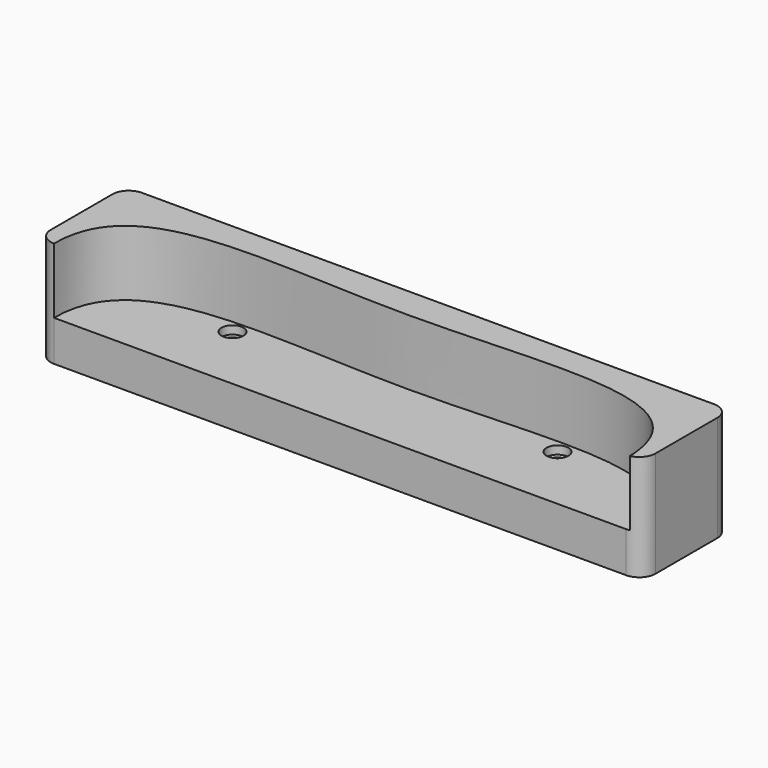
from build123d import *

# Parameters (mm, degrees)
F1_DEPTH = 32.4
F3_DEPTH = 20
F4_R     = 3.35
F5_DEPTH = 2.5
F6_R     = 1.93
F7_DEPTH = 25
F8_R     = 1.93
F9_DEPTH = 25


# Not quite as in the source:
# - a feature names something its author has since deleted; it is built from what else it names


with BuildPart() as f1:
    # F0 (on Top) → F1 (new body)
    with BuildSketch(Plane.XY):
        with BuildLine():
            Line((85.6374964118, -7.5007802074), (-89.3625035882, -7.5007802074))
            ThreePointArc((-89.3625035882, -7.5007802074), (-92.8980374941, -8.9652463014), (-94.3625035882, -12.5007802074))
            Line((-94.3625035882, -12.5007802074), (-94.3625035882, -36.1007802074))
            ThreePointArc((-94.3625035882, -36.1007802074), (-92.8980374941, -39.6363141133), (-89.3625035882, -41.1007802074))
            add(Edge.make_bspline(
                [(-89.3625035882, -41.1007802074), (-59.4269413323, -34.6411043009), (-0.064704069, -1.5309018726), (57.2335608059, -34.7243234216), (85.6374964118, -41.1007802074)],
                knots=[0, 0, 0, 0, 0.5049781057, 1, 1, 1, 1], degree=3))
            ThreePointArc((85.6374964118, -41.1007802074), (89.1730303177, -39.6363141133), (90.6374964118, -36.1007802074))
            Line((90.6374964118, -36.1007802074), (90.6374964118, -12.5007802074))
            ThreePointArc((90.6374964118, -12.5007802074), (89.1730303177, -8.9652463014), (85.6374964118, -7.5007802074))
        make_face()
        with BuildLine():
            add(Edge.make_bspline(
                [(-89.3625035882, -41.1007802074), (-59.4269413323, -34.6411043009), (-0.064704069, -1.5309018726), (57.2335608059, -34.7243234216), (85.6374964118, -41.1007802074)],
                knots=[0, 0, 0, 0, 0.5049781057, 1, 1, 1, 1], degree=3))
            Line((-89.3625035882, -41.1007802074), (85.6374964118, -41.1007802074))
        make_face()
    extrude(amount=F1_DEPTH)

    # F2 (on face) → F3 (cut)
    with BuildSketch(Plane.XY.offset(32.4)):
        with BuildLine():
            add(Edge.make_bspline(
                [(-89.3625035882, -41.1007802074), (-89.3625035882, -7.5007802074), (0.6047339491, -26.7707217669), (85.6374964118, -7.5007802074), (86.6746914089, -40.9920199825)],
                knots=[0, 0, 0, 0, 0.5035939918, 1, 1, 1, 1], degree=3))
            Line((-89.3625035882, -41.1007802074), (85.6374964118, -41.1007802074))
            ThreePointArc((85.6374964118, -41.1007802074), (86.1589372638, -41.0735158165), (86.6746914089, -40.9920199825))
        make_face()
    extrude(amount=-F3_DEPTH, mode=Mode.SUBTRACT)

    # F4 (on face) → F5 (cut)
    with BuildSketch(Plane.XY.offset(12.4)):
        with Locations((-51.5625035882, -20.1007802074)):
            Circle(F4_R)
        with BuildLine():
            ThreePointArc((51.1874964118, -20.1007802074), (47.8374964118, -16.7507802074), (44.4874964118, -20.1007802074))
            ThreePointArc((44.4874964118, -20.1007802074), (47.8374964118, -23.4507802074), (51.1874964118, -20.1007802074))
        make_face()
    extrude(amount=-F5_DEPTH, mode=Mode.SUBTRACT)

    # F6 (on face) → F7 (cut)
    with BuildSketch(Plane.XY.offset(9.9)):
        with Locations((-51.5625035882, -20.1007802074)):
            Circle(F6_R)
    extrude(amount=-F7_DEPTH, mode=Mode.SUBTRACT)

    # F8 (on face) → F9 (cut)
    with BuildSketch(Plane.XY.offset(9.9)):
        with Locations((47.8374964118, -20.1007802074)):
            Circle(F8_R)
    extrude(amount=-F9_DEPTH, mode=Mode.SUBTRACT)


solid = f1.part
